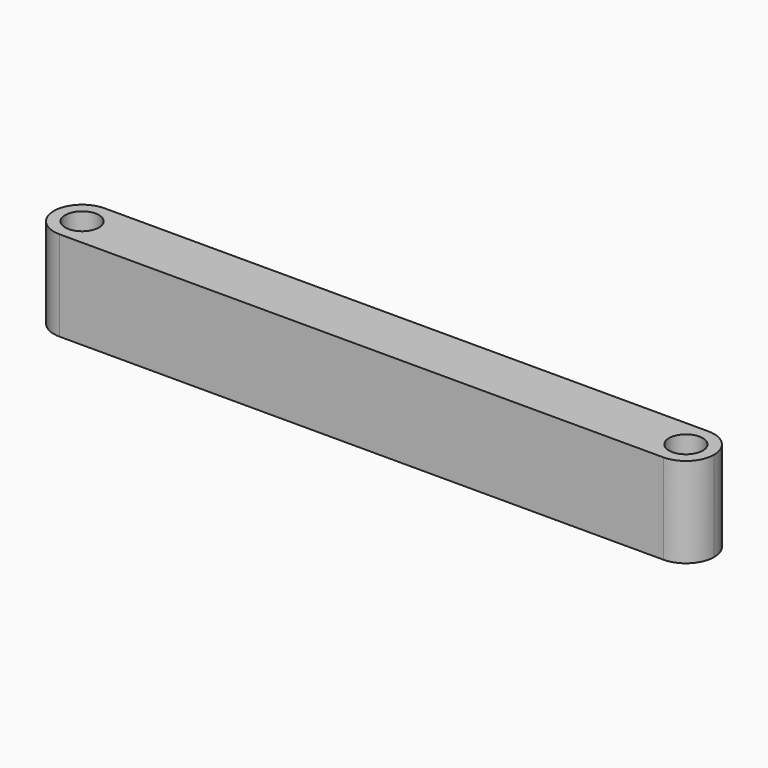
from build123d import *

# Parameters (mm, degrees)
F0_W     = 186.055
F0_H     = 15.875
F1_DEPTH = 25.4
F2_R     = 7.93749
F4_D     = 9.525


# Not quite as in the source:
# - a fillet or chamfer is up to 0.001 mm smaller than in the source, because OpenCascade refuses the exact size


with BuildPart() as f1:
    # F0 (on Top) → F1 (new body)
    with BuildSketch(Plane.XY):
        Rectangle(F0_W, F0_H)
    extrude(amount=F1_DEPTH)

    # F2 (radius 7.9375 in the source; OpenCascade refuses exactly that, so slightly less here)
    f2_edges = [f1.edges().sort_by_distance(p)[0] for p in [
        (-93.0275, -7.9375, 12.7),
        (-93.0275, 7.9375, 12.7),
        (93.0275, -7.9375, 12.7),
        (93.0275, 7.9375, 12.7),
    ]]
    fillet(f2_edges, radius=F2_R)

    # F4 (through all)
    with Locations(Plane.XY.offset(25.4)):
        with Locations((-85.09, 0), (85.09, 0)):
            Hole(F4_D / 2)


solid = f1.part
